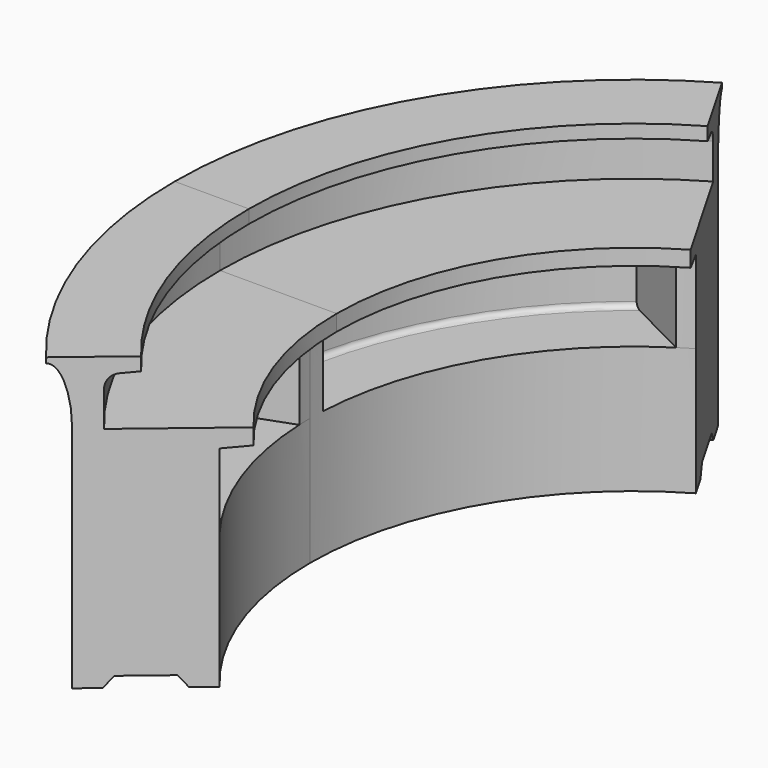
from build123d import *

# Parameters (mm, degrees)
F2_ANGLE = 60
F5_DEPTH = 311.2511336474
F6_ANGLE = 40
F8_DEPTH = 311.2511336474


with BuildPart() as f2:
    # F0 (on Front) → F2 (revolve)
    with BuildSketch(Plane.XZ):
        with BuildLine():
            Line((77, 860), (77, 0))
            Line((77, 0), (167, 0))
            Line((167, 0), (200.5639852471, 40))
            Line((200.5639852471, 40), (387.3966058859, 40))
            Line((387.3966058859, 40), (420.960591133, 0))
            Line((420.960591133, 0), (510.960591133, 0))
            Line((510.960591133, 0), (510.960591133, 480))
            Line((510.960591133, 480), (280.960591133, 480))
            ThreePointArc((280.960591133, 480), (266.8184555093, 485.8578643763), (260.960591133, 500))
            Line((260.960591133, 500), (260.960591133, 751.0523442856))
            ThreePointArc((260.960591133, 751.0523442856), (266.2150443968, 764.5641484379), (279.2174762781, 770.9762382474))
            Line((279.2174762781, 770.9762382474), (610.960591133, 800))
            Line((610.960591133, 800), (610.960591133, 860))
            Line((610.960591133, 860), (170.960591133, 860))
            Line((170.960591133, 860), (170.960591133, 994.6437291457))
            ThreePointArc((170.960591133, 994.6437291457), (184.0967242925, 1028.4232395265), (216.6028039956, 1044.4534640503))
            Line((216.6028039956, 1044.4534640503), (280, 1050))
            Line((280, 1050), (280, 1100))
            Line((280, 1100), (0, 1100))
            Line((0, 1100), (0, 1080))
            add(Edge.make_bspline(
                [(77, 860), (77, 1080), (0, 1080)],
                knots=[4.7123889804, 4.7123889804, 4.7123889804, 6.2831853072, 6.2831853072, 6.2831853072], degree=2, weights=[1, 0.7071067812, 1]))
        make_face()
    revolve(axis=Axis((1730, 0, 0), (0, 0, -1)), revolution_arc=F2_ANGLE)

    # F4 (on face) → F5 (join, through all)
    with BuildSketch(Plane.XY.offset(480)):
        with BuildLine():
            ThreePointArc((510.960591133, 0), (511.3132112784, 29.3187886209), (512.3708677163, 58.6206156975))
            Line((512.3708677163, 58.6206156975), (276.3251008291, 211.9105290561))
            ThreePointArc((276.3251008291, 211.9105290561), (264.8067534678, 106.2333992714), (260.960591133, 0))
            Line((260.960591133, 0), (510.960591133, 0))
        make_face()
        with BuildLine():
            Line((819.6426489226, 1152.9641269977), (1070.4184914786, 1025.187453097))
            ThreePointArc((1070.4184914786, 1025.187453097), (1095.2657898853, 1040.7543239789), (1120.4802955665, 1055.7190962932))
            Line((1120.4802955665, 1055.7190962932), (995.4802955665, 1272.2254472393))
            ThreePointArc((995.4802955665, 1272.2254472393), (905.4025542345, 1215.7778733146), (819.6426489226, 1152.9641269977))
        make_face()
    extrude(amount=F5_DEPTH)


with BuildPart() as f6:
    # F0 (on Front) → F6 (revolve)
    with BuildSketch(Plane.XZ):
        with BuildLine():
            Line((77, 860), (77, 0))
            Line((77, 0), (167, 0))
            Line((167, 0), (200.5639852471, 40))
            Line((200.5639852471, 40), (387.3966058859, 40))
            Line((387.3966058859, 40), (420.960591133, 0))
            Line((420.960591133, 0), (510.960591133, 0))
            Line((510.960591133, 0), (510.960591133, 480))
            Line((510.960591133, 480), (280.960591133, 480))
            ThreePointArc((280.960591133, 480), (266.8184555093, 485.8578643763), (260.960591133, 500))
            Line((260.960591133, 500), (260.960591133, 751.0523442856))
            ThreePointArc((260.960591133, 751.0523442856), (266.2150443968, 764.5641484379), (279.2174762781, 770.9762382474))
            Line((279.2174762781, 770.9762382474), (610.960591133, 800))
            Line((610.960591133, 800), (610.960591133, 860))
            Line((610.960591133, 860), (170.960591133, 860))
            Line((170.960591133, 860), (170.960591133, 994.6437291457))
            ThreePointArc((170.960591133, 994.6437291457), (184.0967242925, 1028.4232395265), (216.6028039956, 1044.4534640503))
            Line((216.6028039956, 1044.4534640503), (280, 1050))
            Line((280, 1050), (280, 1100))
            Line((280, 1100), (0, 1100))
            Line((0, 1100), (0, 1080))
            add(Edge.make_bspline(
                [(77, 860), (77, 1080), (0, 1080)],
                knots=[4.7123889804, 4.7123889804, 4.7123889804, 6.2831853072, 6.2831853072, 6.2831853072], degree=2, weights=[1, 0.7071067812, 1]))
        make_face()
    revolve(axis=Axis((1730, 0, 0), (0, 0, 1)), revolution_arc=F6_ANGLE)

    # F7 (on face) → F8 (join, through all)
    with BuildSketch(Plane.XY.offset(480)):
        with BuildLine():
            ThreePointArc((518.8103838976, -831.3221389148), (560.36603147, -888.838098005), (604.6505241146, -944.2803301609))
            Line((604.6505241146, -944.2803301609), (796.1616348944, -783.5834277393))
            ThreePointArc((796.1616348944, -783.5834277393), (779.4094834165, -763.1741283301), (763.1032953401, -742.4067907075))
            Line((763.1032953401, -742.4067907075), (518.8103838976, -831.3221389148))
        make_face()
        with BuildLine():
            Line((267.8113544688, -141.7079732541), (512.1042659113, -52.7926250468))
            ThreePointArc((512.1042659113, -52.7926250468), (511.2465433657, -26.4025058059), (510.960591133, 0))
            Line((510.960591133, 0), (260.960591133, 0))
            ThreePointArc((260.960591133, 0), (262.6742815095, -70.9367370304), (267.8113544688, -141.7079732541))
        make_face()
    extrude(amount=F8_DEPTH)


solid = Compound([f2.part, f6.part])
